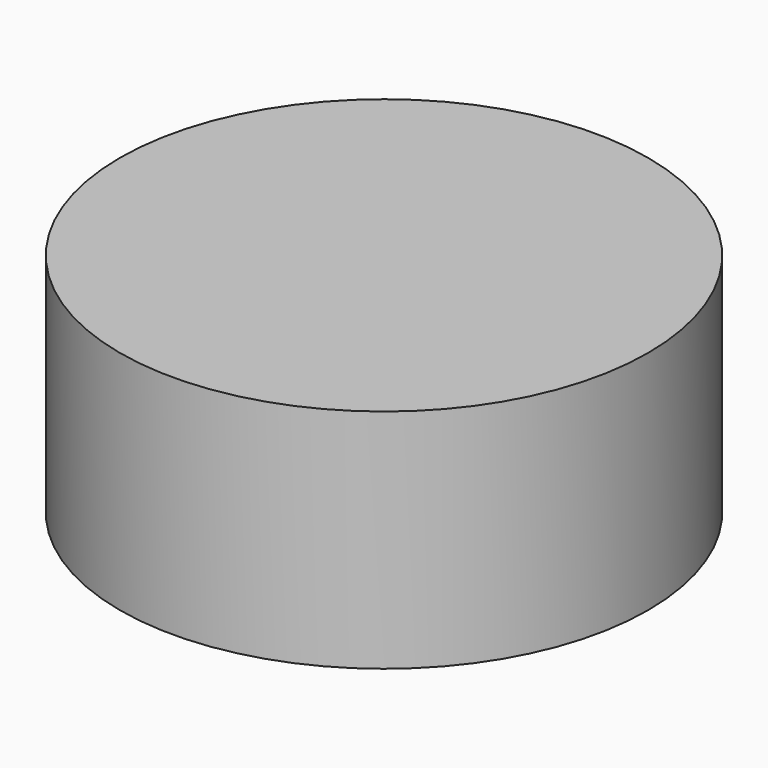
from build123d import *

# Parameters (mm, degrees)
F0_R     = 29.1547594742
F1_DEPTH = 25


# Not quite as in the source:
# - a feature of the source that left no trace in its solid (it failed there, or was rolled back) is left out


with BuildPart() as f1:
    # F0 (on Top) → F1 (new body)
    with BuildSketch(Plane.XY):
        with Locations((-25, 15)):
            Circle(F0_R)
    extrude(amount=F1_DEPTH)


solid = f1.part
